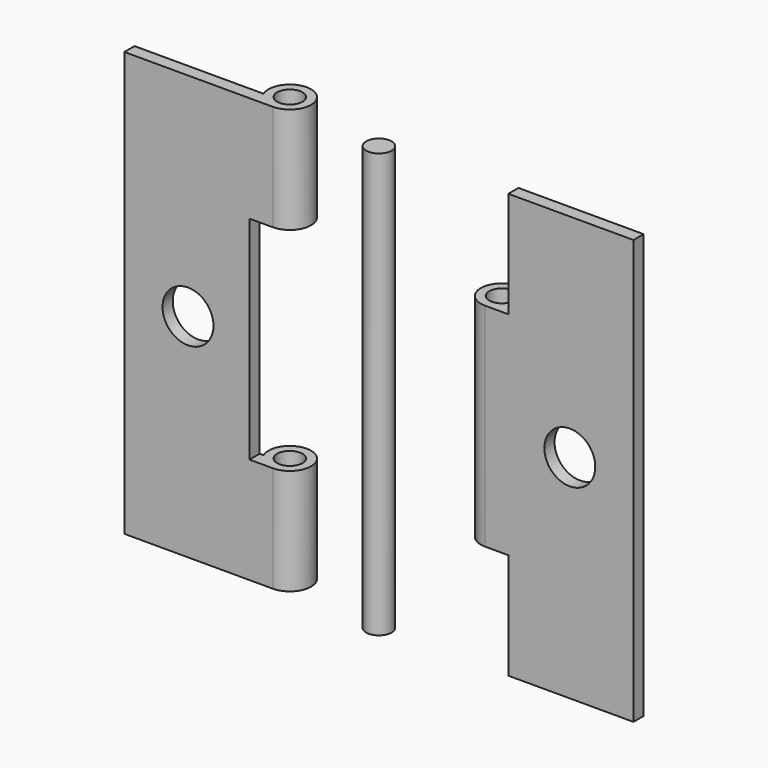
from build123d import *

# Parameters (mm, degrees)
F1_R      = 5
F1_R_2    = 3
F2_DEPTH  = 50
F4_W      = 3
F4_H      = 100
F0_R      = 6
F6_DEPTH  = 3
F0_W      = 5.5
F0_H      = 50
F7_DEPTH  = 11
F10_R     = 5
F10_R_2   = 3
F11_DEPTH = 50
F13_W     = 3
F13_H     = 100
F9_R      = 6
F15_DEPTH = 3
F9_W      = 5.5
F9_H      = 25
F16_DEPTH = 11
F18_R     = 3
F19_DEPTH = 50


with BuildPart() as f2:
    # F1 (on Top) → F2 (new body, symmetric)
    with BuildSketch(Plane.XY):
        with Locations((0, 5)):
            Circle(F1_R)
        with Locations((0, 5)):
            Circle(F1_R_2, mode=Mode.SUBTRACT)
    extrude(amount=F2_DEPTH, both=True)

    # F4 (on offset) → F5 (join, up to the next surface of F2)
    with BuildSketch(Plane.YZ.offset(-35)):
        with Locations((1.5, 0)):
            Rectangle(F4_W, F4_H)
    extrude(until=Until.NEXT)

    # F0 (on Front) → F6 (cut, through all)
    with BuildSketch(Plane.XZ):
        with Locations((-20, 0)):
            Circle(F0_R)
    extrude(amount=-F6_DEPTH, mode=Mode.SUBTRACT)

    # F0 (on Front) → F7 (cut)
    with BuildSketch(Plane.XZ):
        with Locations((2.75, 0)):
            Rectangle(F0_W, F0_H)
        with Locations((-2.75, 0)):
            Rectangle(F0_W, F0_H)
    extrude(amount=-F7_DEPTH, mode=Mode.SUBTRACT)


with BuildPart() as f11:
    # F10 (on Top) → F11 (new body, symmetric)
    with BuildSketch(Plane.XY):
        with Locations((50.0151987175, 4.9999768998)):
            Circle(F10_R)
        with Locations((50.0151987175, 4.9999768998)):
            Circle(F10_R_2, mode=Mode.SUBTRACT)
    extrude(amount=F11_DEPTH, both=True)

    # F13 (on offset) → F14 (join, up to the next surface of F11)
    with BuildSketch(Plane.YZ.offset(85)):
        with Locations((1.5, 0)):
            Rectangle(F13_W, F13_H)
    extrude(until=Until.NEXT, dir=(-1, 0, 0))

    # F9 (on Front) → F15 (cut, through all)
    with BuildSketch(Plane.XZ):
        with Locations((70, 0)):
            Circle(F9_R)
    extrude(amount=-F15_DEPTH, mode=Mode.SUBTRACT)

    # F9 (on Front) → F16 (cut)
    with BuildSketch(Plane.XZ):
        with Locations((47.25, -37.5)):
            Rectangle(F9_W, F9_H)
        with Locations((47.25, 37.5)):
            Rectangle(F9_W, F9_H)
        with Locations((52.75, 37.5)):
            Rectangle(F9_W, F9_H)
        with Locations((52.75, -37.5)):
            Rectangle(F9_W, F9_H)
    extrude(amount=-F16_DEPTH, mode=Mode.SUBTRACT)


with BuildPart() as f19:
    # F18 (on Top) → F19 (new body, symmetric)
    with BuildSketch(Plane.XY):
        with Locations((25, 0)):
            Circle(F18_R)
    extrude(amount=F19_DEPTH, both=True)


solid = Compound([f2.part, f11.part, f19.part])
